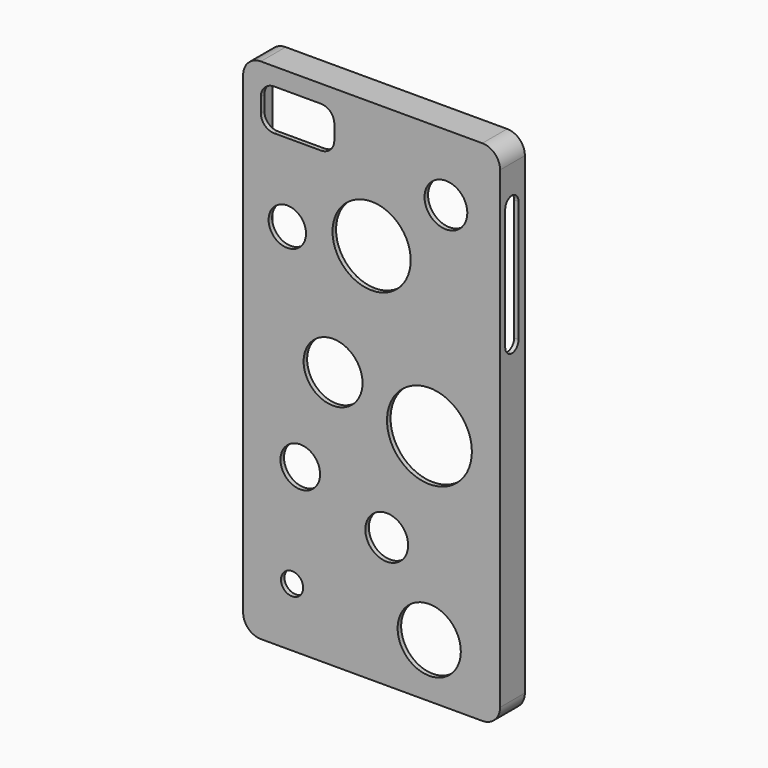
from build123d import *

# Parameters (mm, degrees)
F0_W         = 73.66
F0_H         = 145.796
F1_DEPTH     = 8.89
F2_R         = 5.08
F3_W         = 21.0629868459
F3_H         = 11.8066714083
F4_DEPTH     = 12.7
F5_R         = 3.81
F7_T         = -1.27
F9_DEPTH     = 7.62
F10_W        = 4.164762795
F10_H        = 13.3272446692
F11_DEPTH    = 25.4
F12_T1_DEPTH = 1.27
F13_W        = 57.5663968921
F13_H        = 5.6068669073
F14_DEPTH    = 25.4
F15_R        = 2.54
F16_W        = 4.7923256643
F16_H        = 39.9060079362
F17_DEPTH    = 25.4
F18_T1_DEPTH = 1.27
F20_DEPTH    = 25.4
F21_R        = 12.1645390549
F21_R_2      = 8.4445659424
F21_R_3      = 5.6782177744
F21_R_4      = 6.1332477191
F21_R_5      = 9.0595333528
F21_R_6      = 3.1849618728
F21_R_7      = 5.3665907278
F21_R_8      = 6.1379255293
F22_DEPTH    = 25.4


# Not quite as in the source:
# - a fillet or chamfer that OpenCascade refuses, or shapes differently, is made with other operations: its cross-section is extruded or revolved along the edge and cut away or added


with BuildPart() as f1:
    # F0 (on Front) → F1 (new body)
    with BuildSketch(Plane.XZ):
        with Locations((-5.763799886, -17.0958732503)):
            Rectangle(F0_W, F0_H)
    extrude(amount=F1_DEPTH)

    # F2
    f2_edges = [f1.edges().sort_by_distance(p)[0] for p in [
        (31.0662, -4.445, 55.802127),
        (-42.5938, -4.445, 55.802127),
        (31.0662, -4.445, -89.993873),
        (-42.5938, -4.445, -89.993873),
    ]]
    fillet(f2_edges, radius=F2_R)

    # F3 (on face) → F4 (cut, symmetric)
    with BuildSketch(Plane.XZ.offset(8.89)):
        with Locations((-26.9823064631, 44.8187910455)):
            Rectangle(F3_W, F3_H)
    extrude(amount=F4_DEPTH, both=True, mode=Mode.SUBTRACT)

    # F5
    f5_edges = [f1.edges().sort_by_distance(p)[0] for p in [
        (-16.450813, -4.445, 50.722127),
        (-37.5138, -4.445, 50.722127),
        (-37.5138, -4.445, 38.915455),
        (-16.450813, -4.445, 38.915455),
    ]]
    fillet(f5_edges, radius=F5_R)

    # F7
    f7_openings = [f1.faces().sort_by_distance(p)[0] for p in [
        (-5.285571, 0, -18.491325),
    ]]
    offset(amount=F7_T, openings=f7_openings)

    # F8 (on face) → F9 (cut)
    with BuildSketch(Plane(origin=(0, 0, 0), x_dir=(-1, 0, 0), z_dir=(0, 1, 0))):
        Polygon((23.2353508472, 53.487226367), (11.2448604777, 51.826223731), (11.2448604777, 31.8353585899), (37.2746288776, 33.5012637079), (40.1331484318, 42.7181646228), (38.7322939932, 52.0863756537), align=None)
    extrude(amount=-F9_DEPTH, mode=Mode.SUBTRACT)

    # F10 (on face) → F11 (cut)
    with BuildSketch(Plane(origin=(-42.593799886, 0, 0), x_dir=(0, -1, 0), z_dir=(-1, 0, 0))):
        with Locations((4.5812404715, 30.585931614)):
            Rectangle(F10_W, F10_H)
    extrude(amount=-F11_DEPTH, mode=Mode.SUBTRACT)

    # F12: fillet of radius 2.54 on 4 edges, made by hand

    # F12_s2 → F12_t1 (join)
    with BuildSketch(Plane.YZ.offset(-42.593799886)):
        with BuildLine():
            ThreePointArc((-6.6636218689, 34.7095539486), (-5.9196730932, 36.5056051729), (-4.1236218689, 37.2495539486))
            Line((-4.1236218689, 37.2495539486), (-6.6636218689, 37.2495539486))
            Line((-6.6636218689, 37.2495539486), (-6.6636218689, 34.7095539486))
        make_face()
        with BuildLine():
            ThreePointArc((-6.6636218689, 26.4623092794), (-5.9196730932, 24.6662580552), (-4.1236218689, 23.9223092794))
            Line((-4.1236218689, 23.9223092794), (-6.6636218689, 23.9223092794))
            Line((-6.6636218689, 23.9223092794), (-6.6636218689, 26.4623092794))
        make_face()
        with BuildLine():
            ThreePointArc((-2.498859074, 34.7095539486), (-3.2428078498, 36.5056051729), (-5.038859074, 37.2495539486))
            Line((-5.038859074, 37.2495539486), (-2.498859074, 37.2495539486))
            Line((-2.498859074, 37.2495539486), (-2.498859074, 34.7095539486))
        make_face()
        with BuildLine():
            ThreePointArc((-5.038859074, 23.9223092794), (-3.2428078498, 24.6662580552), (-2.498859074, 26.4623092794))
            Line((-2.498859074, 26.4623092794), (-2.498859074, 23.9223092794))
            Line((-2.498859074, 23.9223092794), (-5.038859074, 23.9223092794))
        make_face()
    extrude(amount=F12_T1_DEPTH)

    # F13 (on face) → F14 (cut)
    with BuildSketch(Plane(origin=(0, 0, -89.9938732503), x_dir=(1, 0, 0), z_dir=(0, 0, -1))):
        with Locations((-5.0962045789, 4.3330059852)):
            Rectangle(F13_W, F13_H)
    extrude(amount=-F14_DEPTH, mode=Mode.SUBTRACT)

    # F15
    f15_edges = [f1.edges().sort_by_distance(p)[0] for p in [
        (-33.879403, -7.136439, -89.358873),
        (23.686994, -7.136439, -89.358873),
        (-33.879403, -1.529573, -89.358873),
        (23.686994, -1.529573, -89.358873),
    ]]
    fillet(f15_edges, radius=F15_R)

    # F16 (on face) → F17 (cut)
    with BuildSketch(Plane.YZ.offset(31.066200114)):
        with Locations((-4.6495434362, 22.6213793503)):
            Rectangle(F16_W, F16_H)
    extrude(amount=-F17_DEPTH, mode=Mode.SUBTRACT)

    # F18: fillet of radius 2.54 on 4 edges, made by hand

    # F18_s2 → F18_t1 (join)
    with BuildSketch(Plane.YZ.offset(29.796200114)):
        with BuildLine():
            ThreePointArc((-4.7933806041, 42.5743833184), (-2.9973293799, 41.8304345426), (-2.2533806041, 40.0343833184))
            Line((-2.2533806041, 40.0343833184), (-2.2533806041, 42.5743833184))
            Line((-2.2533806041, 42.5743833184), (-4.7933806041, 42.5743833184))
        make_face()
        with BuildLine():
            ThreePointArc((-2.2533806041, 5.2083753822), (-2.9973293799, 3.412324158), (-4.7933806041, 2.6683753822))
            Line((-4.7933806041, 2.6683753822), (-2.2533806041, 2.6683753822))
            Line((-2.2533806041, 2.6683753822), (-2.2533806041, 5.2083753822))
        make_face()
        with BuildLine():
            ThreePointArc((-4.5057062684, 42.5743833184), (-6.3017574926, 41.8304345426), (-7.0457062684, 40.0343833184))
            Line((-7.0457062684, 40.0343833184), (-7.0457062684, 42.5743833184))
            Line((-7.0457062684, 42.5743833184), (-4.5057062684, 42.5743833184))
        make_face()
        with BuildLine():
            ThreePointArc((-4.5057062684, 2.6683753822), (-6.3017574926, 3.412324158), (-7.0457062684, 5.2083753822))
            Line((-7.0457062684, 5.2083753822), (-7.0457062684, 2.6683753822))
            Line((-7.0457062684, 2.6683753822), (-4.5057062684, 2.6683753822))
        make_face()
    extrude(amount=F18_T1_DEPTH)

    # F19 (on face) → F20 (cut)
    with BuildSketch(Plane.XZ.offset(8.89)):
        with BuildLine():
            Line((-5.763799886, 8.3429517969), (-5.763799886, 30.7556648925))
            ThreePointArc((-5.763799886, 30.7556648925), (-16.9701564338, 19.5493083447), (-5.763799886, 8.3429517969))
        make_face()
        with BuildLine():
            ThreePointArc((5.4425566618, 19.5493083447), (2.1602908213, 27.473399052), (-5.763799886, 30.7556648925))
            Line((-5.763799886, 30.7556648925), (-5.763799886, 8.3429517969))
            ThreePointArc((-5.763799886, 8.3429517969), (2.1602908213, 11.6252176374), (5.4425566618, 19.5493083447))
        make_face()
    extrude(amount=-F20_DEPTH, mode=Mode.SUBTRACT)

    # F21 (on face) → F22 (cut)
    with BuildSketch(Plane.XZ.offset(8.89)):
        with Locations((10.8195273206, -23.030474782)):
            Circle(F21_R)
        with Locations((-16.8110914528, -15.915196389)):
            Circle(F21_R_2)
        with Locations((-26.2109395117, -42.8681261837)):
            Circle(F21_R_3)
        with Locations((-1.4226717176, -52.5855049491)):
            Circle(F21_R_4)
        with Locations((10.7564115897, -74.5054781437)):
            Circle(F21_R_5)
        with Locations((-28.563728556, -73.1163173914)):
            Circle(F21_R_6)
        with Locations((-29.9305599183, 16.5542345494)):
            Circle(F21_R_7)
        with Locations((15.5416298658, 36.8061438203)):
            Circle(F21_R_8)
    extrude(amount=-F22_DEPTH, mode=Mode.SUBTRACT)


solid = f1.part
